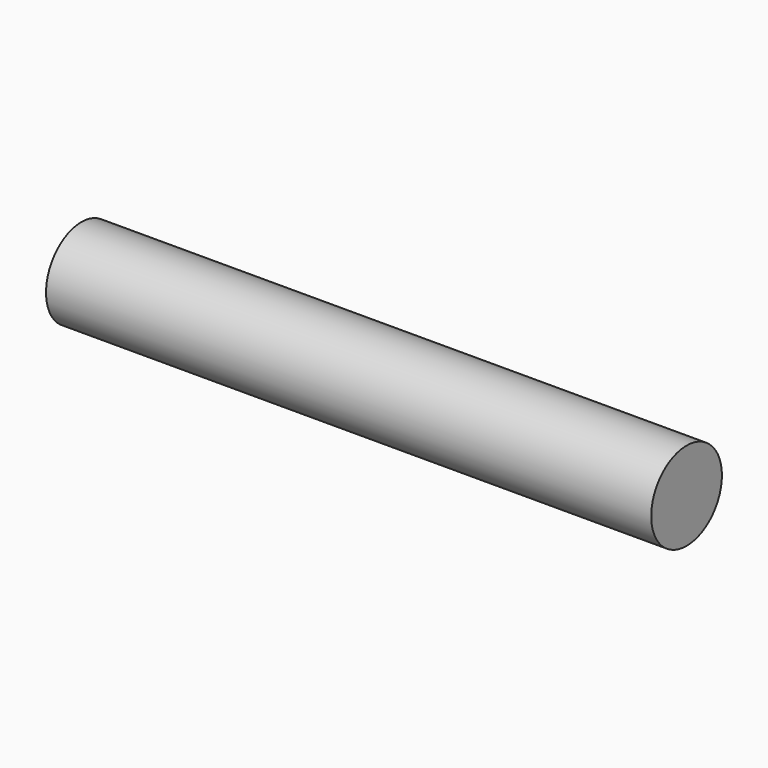
from build123d import *

# Parameters (mm, degrees)
F0_R     = 4.6374466258
F2_DEPTH = 63.5


# Not quite as in the source:
# - the program builds the solid bodies; features that only make, move or delete a surface that nothing else refers to are left out


with BuildPart() as f2:
    # F0 (on Right) → F2 (new body)
    with BuildSketch(Plane.YZ):
        Circle(F0_R)
    extrude(amount=F2_DEPTH)


solid = f2.part
